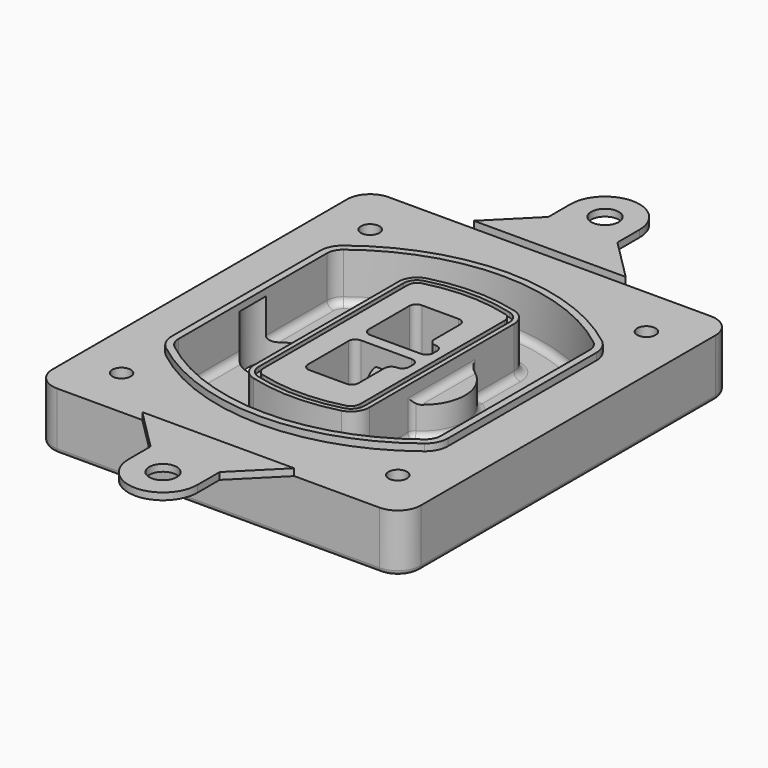
from build123d import *

# Parameters (mm, degrees)
F0_R      = 4
F1_DEPTH  = 25
F2_DEPTH  = 3
F3_DEPTH  = 18
F5_DEPTH  = 21
F6_DEPTH  = 2
F8_DEPTH  = 20
F9_DEPTH  = 16
F10_DEPTH = 25
F7_R      = 6
F7_R_2    = 4
F11_DEPTH = 6
F13_DEPTH = 9
F14_R     = 3
F15_R     = 2
F16_R     = 6
F17_DEPTH = 3


# Not quite as in the source:
# - a feature names something its author has since deleted; it is built from what else it names


with BuildPart() as f1:
    # F0 (on Top) → F1 (new body)
    with BuildSketch(Plane.XY):
        with BuildLine():
            ThreePointArc((-80, -80), (-77.0710678119, -87.0710678119), (-70, -90))
            Line((-70, -90), (70, -90))
            ThreePointArc((70, -90), (77.0710678119, -87.0710678119), (80, -80))
            Line((80, -80), (80, 80))
            ThreePointArc((80, 80), (77.0710678119, 87.0710678119), (70, 90))
            Line((70, 90), (-70, 90))
            ThreePointArc((-70, 90), (-77.0710678119, 87.0710678119), (-80, 80))
            Line((-80, 80), (-80, -80))
        make_face()
        with Locations((-60, -67.5)):
            Circle(F0_R, mode=Mode.SUBTRACT)
        with Locations((60, -67.5)):
            Circle(F0_R, mode=Mode.SUBTRACT)
        with Locations((-60, 67.5)):
            Circle(F0_R, mode=Mode.SUBTRACT)
        with BuildLine():
            ThreePointArc((-64, 40.2934422872), (-62.5820384798, 46.4328484224), (-58.6153846154, 51.3286200352))
            ThreePointArc((-58.6153846154, 51.3286200352), (0, 71.5), (58.6153846154, 51.3286200352))
            ThreePointArc((58.6153846154, 51.3286200352), (62.5820384798, 46.4328484224), (64, 40.2934422872))
            Line((64, 40.2934422872), (64, -40.2934422872))
            ThreePointArc((64, -40.2934422872), (62.5820384798, -46.4328484224), (58.6153846154, -51.3286200352))
            ThreePointArc((58.6153846154, -51.3286200352), (0, -71.5), (-58.6153846154, -51.3286200352))
            ThreePointArc((-58.6153846154, -51.3286200352), (-62.5820384798, -46.4328484224), (-64, -40.2934422872))
            Line((-64, -40.2934422872), (-64, 40.2934422872))
        make_face(mode=Mode.SUBTRACT)
        with Locations((60, 67.5)):
            Circle(F0_R, mode=Mode.SUBTRACT)
        with BuildLine():
            ThreePointArc((58.6153846154, 51.3286200352), (0, 71.5), (-58.6153846154, 51.3286200352))
            ThreePointArc((-58.6153846154, 51.3286200352), (-62.5820384798, 46.4328484224), (-64, 40.2934422872))
            Line((-64, 40.2934422872), (-64, -40.2934422872))
            ThreePointArc((-64, -40.2934422872), (-62.5820384798, -46.4328484224), (-58.6153846154, -51.3286200352))
            ThreePointArc((-58.6153846154, -51.3286200352), (0, -71.5), (58.6153846154, -51.3286200352))
            ThreePointArc((58.6153846154, -51.3286200352), (62.5820384798, -46.4328484224), (64, -40.2934422872))
            Line((64, -40.2934422872), (64, 40.2934422872))
            ThreePointArc((64, 40.2934422872), (62.5820384798, 46.4328484224), (58.6153846154, 51.3286200352))
        make_face()
        with BuildLine():
            Line((-60, -40.2934422872), (-60, 40.2934422872))
            ThreePointArc((-60, 40.2934422872), (-58.9871703427, 44.6787323838), (-56.1538461538, 48.1757121072))
            ThreePointArc((-56.1538461538, 48.1757121072), (0, 67.5), (56.1538461538, 48.1757121072))
            ThreePointArc((56.1538461538, 48.1757121072), (58.9871703427, 44.6787323838), (60, 40.2934422872))
            Line((60, 40.2934422872), (60, -40.2934422872))
            ThreePointArc((60, -40.2934422872), (58.9871703427, -44.6787323838), (56.1538461538, -48.1757121072))
            ThreePointArc((56.1538461538, -48.1757121072), (0, -67.5), (-56.1538461538, -48.1757121072))
            ThreePointArc((-56.1538461538, -48.1757121072), (-58.9871703427, -44.6787323838), (-60, -40.2934422872))
        make_face(mode=Mode.SUBTRACT)
        with BuildLine():
            ThreePointArc((-56.1538461538, 48.1757121072), (-58.9871703427, 44.6787323838), (-60, 40.2934422872))
            Line((-60, 40.2934422872), (-60, -40.2934422872))
            ThreePointArc((-60, -40.2934422872), (-58.9871703427, -44.6787323838), (-56.1538461538, -48.1757121072))
            ThreePointArc((-56.1538461538, -48.1757121072), (0, -67.5), (56.1538461538, -48.1757121072))
            ThreePointArc((56.1538461538, -48.1757121072), (58.9871703427, -44.6787323838), (60, -40.2934422872))
            Line((60, -40.2934422872), (60, 40.2934422872))
            ThreePointArc((60, 40.2934422872), (58.9871703427, 44.6787323838), (56.1538461538, 48.1757121072))
            ThreePointArc((56.1538461538, 48.1757121072), (0, 67.5), (-56.1538461538, 48.1757121072))
        make_face()
        with BuildLine():
            ThreePointArc((54.3076923077, 45.8110311612), (56.2910192399, 43.3631453548), (57, 40.2934422872))
            Line((57, 40.2934422872), (57, -40.2934422872))
            ThreePointArc((57, -40.2934422872), (56.2910192399, -43.3631453548), (54.3076923077, -45.8110311612))
            ThreePointArc((54.3076923077, -45.8110311612), (0, -64.5), (-54.3076923077, -45.8110311612))
            ThreePointArc((-54.3076923077, -45.8110311612), (-56.2910192399, -43.3631453548), (-57, -40.2934422872))
            Line((-57, -40.2934422872), (-57, 40.2934422872))
            ThreePointArc((-57, 40.2934422872), (-56.2910192399, 43.3631453548), (-54.3076923077, 45.8110311612))
            ThreePointArc((-54.3076923077, 45.8110311612), (0, 64.5), (54.3076923077, 45.8110311612))
        make_face(mode=Mode.SUBTRACT)
        with BuildLine():
            Line((57, -40.2934422872), (57, 40.2934422872))
            ThreePointArc((57, 40.2934422872), (56.2910192399, 43.3631453548), (54.3076923077, 45.8110311612))
            ThreePointArc((54.3076923077, 45.8110311612), (0, 64.5), (-54.3076923077, 45.8110311612))
            ThreePointArc((-54.3076923077, 45.8110311612), (-56.2910192399, 43.3631453548), (-57, 40.2934422872))
            Line((-57, 40.2934422872), (-57, -40.2934422872))
            ThreePointArc((-57, -40.2934422872), (-56.2910192399, -43.3631453548), (-54.3076923077, -45.8110311612))
            ThreePointArc((-54.3076923077, -45.8110311612), (0, -64.5), (54.3076923077, -45.8110311612))
            ThreePointArc((54.3076923077, -45.8110311612), (56.2910192399, -43.3631453548), (57, -40.2934422872))
        make_face()
    extrude(amount=-F1_DEPTH)

    # F0 (on Top) → F2 (join)
    with BuildSketch(Plane.XY):
        with BuildLine():
            ThreePointArc((-56.1538461538, 48.1757121072), (-58.9871703427, 44.6787323838), (-60, 40.2934422872))
            Line((-60, 40.2934422872), (-60, -40.2934422872))
            ThreePointArc((-60, -40.2934422872), (-58.9871703427, -44.6787323838), (-56.1538461538, -48.1757121072))
            ThreePointArc((-56.1538461538, -48.1757121072), (0, -67.5), (56.1538461538, -48.1757121072))
            ThreePointArc((56.1538461538, -48.1757121072), (58.9871703427, -44.6787323838), (60, -40.2934422872))
            Line((60, -40.2934422872), (60, 40.2934422872))
            ThreePointArc((60, 40.2934422872), (58.9871703427, 44.6787323838), (56.1538461538, 48.1757121072))
            ThreePointArc((56.1538461538, 48.1757121072), (0, 67.5), (-56.1538461538, 48.1757121072))
        make_face()
        with BuildLine():
            ThreePointArc((54.3076923077, 45.8110311612), (56.2910192399, 43.3631453548), (57, 40.2934422872))
            Line((57, 40.2934422872), (57, -40.2934422872))
            ThreePointArc((57, -40.2934422872), (56.2910192399, -43.3631453548), (54.3076923077, -45.8110311612))
            ThreePointArc((54.3076923077, -45.8110311612), (0, -64.5), (-54.3076923077, -45.8110311612))
            ThreePointArc((-54.3076923077, -45.8110311612), (-56.2910192399, -43.3631453548), (-57, -40.2934422872))
            Line((-57, -40.2934422872), (-57, 40.2934422872))
            ThreePointArc((-57, 40.2934422872), (-56.2910192399, 43.3631453548), (-54.3076923077, 45.8110311612))
            ThreePointArc((-54.3076923077, 45.8110311612), (0, 64.5), (54.3076923077, 45.8110311612))
        make_face(mode=Mode.SUBTRACT)
    extrude(amount=F2_DEPTH)

    # F0 (on Top) → F3 (cut)
    with BuildSketch(Plane.XY):
        with BuildLine():
            Line((57, -40.2934422872), (57, 40.2934422872))
            ThreePointArc((57, 40.2934422872), (56.2910192399, 43.3631453548), (54.3076923077, 45.8110311612))
            ThreePointArc((54.3076923077, 45.8110311612), (0, 64.5), (-54.3076923077, 45.8110311612))
            ThreePointArc((-54.3076923077, 45.8110311612), (-56.2910192399, 43.3631453548), (-57, 40.2934422872))
            Line((-57, 40.2934422872), (-57, -40.2934422872))
            ThreePointArc((-57, -40.2934422872), (-56.2910192399, -43.3631453548), (-54.3076923077, -45.8110311612))
            ThreePointArc((-54.3076923077, -45.8110311612), (0, -64.5), (54.3076923077, -45.8110311612))
            ThreePointArc((54.3076923077, -45.8110311612), (56.2910192399, -43.3631453548), (57, -40.2934422872))
        make_face()
    extrude(amount=-F3_DEPTH, mode=Mode.SUBTRACT)

    # F4 (on face) → F5 (join, through all)
    with BuildSketch(Plane.XY.offset(3)):
        with BuildLine():
            ThreePointArc((-25, -39.2465276821), (-23.3511545998, -44.1109737193), (-19.0842911877, -46.9702398883))
            ThreePointArc((-19.0842911877, -46.9702398883), (0, -49.5), (19.0842911877, -46.9702398883))
            ThreePointArc((19.0842911877, -46.9702398883), (23.3511545998, -44.1109737193), (25, -39.2465276821))
            Line((25, -39.2465276821), (25, 39.2465276821))
            ThreePointArc((25, 39.2465276821), (23.3511545998, 44.1109737193), (19.0842911877, 46.9702398883))
            ThreePointArc((19.0842911877, 46.9702398883), (0, 49.5), (-19.0842911877, 46.9702398883))
            ThreePointArc((-19.0842911877, 46.9702398883), (-23.3511545998, 44.1109737193), (-25, 39.2465276821))
            Line((-25, 39.2465276821), (-25, -39.2465276821))
        make_face()
        with BuildLine():
            ThreePointArc((18.5632183908, 45.0393118368), (21.7633659499, 42.89486221), (23, 39.2465276821))
            Line((23, 39.2465276821), (23, -39.2465276821))
            ThreePointArc((23, -39.2465276821), (21.7633659499, -42.89486221), (18.5632183908, -45.0393118368))
            ThreePointArc((18.5632183908, -45.0393118368), (0, -47.5), (-18.5632183908, -45.0393118368))
            ThreePointArc((-18.5632183908, -45.0393118368), (-21.7633659499, -42.89486221), (-23, -39.2465276821))
            Line((-23, -39.2465276821), (-23, 39.2465276821))
            ThreePointArc((-23, 39.2465276821), (-21.7633659499, 42.89486221), (-18.5632183908, 45.0393118368))
            ThreePointArc((-18.5632183908, 45.0393118368), (0, 47.5), (18.5632183908, 45.0393118368))
        make_face(mode=Mode.SUBTRACT)
        with BuildLine():
            Line((23, -39.2465276821), (23, 39.2465276821))
            ThreePointArc((23, 39.2465276821), (21.7633659499, 42.89486221), (18.5632183908, 45.0393118368))
            ThreePointArc((18.5632183908, 45.0393118368), (0, 47.5), (-18.5632183908, 45.0393118368))
            ThreePointArc((-18.5632183908, 45.0393118368), (-21.7633659499, 42.89486221), (-23, 39.2465276821))
            Line((-23, 39.2465276821), (-23, -39.2465276821))
            ThreePointArc((-23, -39.2465276821), (-21.7633659499, -42.89486221), (-18.5632183908, -45.0393118368))
            ThreePointArc((-18.5632183908, -45.0393118368), (0, -47.5), (18.5632183908, -45.0393118368))
            ThreePointArc((18.5632183908, -45.0393118368), (21.7633659499, -42.89486221), (23, -39.2465276821))
        make_face()
        with BuildLine():
            ThreePointArc((18.0421455939, 43.1083837852), (20.1755772999, 41.6787507007), (21, 39.2465276821))
            Line((21, 39.2465276821), (21, -39.2465276821))
            ThreePointArc((21, -39.2465276821), (20.1755772999, -41.6787507007), (18.0421455939, -43.1083837852))
            ThreePointArc((18.0421455939, -43.1083837852), (0, -45.5), (-18.0421455939, -43.1083837852))
            ThreePointArc((-18.0421455939, -43.1083837852), (-20.1755772999, -41.6787507007), (-21, -39.2465276821))
            Line((-21, -39.2465276821), (-21, 39.2465276821))
            ThreePointArc((-21, 39.2465276821), (-20.1755772999, 41.6787507007), (-18.0421455939, 43.1083837852))
            ThreePointArc((-18.0421455939, 43.1083837852), (0, 45.5), (18.0421455939, 43.1083837852))
        make_face(mode=Mode.SUBTRACT)
        with BuildLine():
            Line((21, -39.2465276821), (21, 39.2465276821))
            ThreePointArc((21, 39.2465276821), (20.1755772999, 41.6787507007), (18.0421455939, 43.1083837852))
            ThreePointArc((18.0421455939, 43.1083837852), (0, 45.5), (-18.0421455939, 43.1083837852))
            ThreePointArc((-18.0421455939, 43.1083837852), (-20.1755772999, 41.6787507007), (-21, 39.2465276821))
            Line((-21, 39.2465276821), (-21, -39.2465276821))
            ThreePointArc((-21, -39.2465276821), (-20.1755772999, -41.6787507007), (-18.0421455939, -43.1083837852))
            ThreePointArc((-18.0421455939, -43.1083837852), (0, -45.5), (18.0421455939, -43.1083837852))
            ThreePointArc((18.0421455939, -43.1083837852), (20.1755772999, -41.6787507007), (21, -39.2465276821))
        make_face()
        with BuildLine():
            Line((-8, -2.5), (14, -2.5))
            ThreePointArc((14, -2.5), (16.1213203436, -3.3786796564), (17, -5.5))
            Line((17, -5.5), (17, -7.5))
            ThreePointArc((17, -7.5), (16.1213203436, -9.6213203436), (14, -10.5))
            ThreePointArc((14, -10.5), (11.8786796564, -11.3786796564), (11, -13.5))
            Line((11, -13.5), (11, -27.5))
            ThreePointArc((11, -27.5), (10.1213203436, -29.6213203436), (8, -30.5))
            Line((8, -30.5), (-8, -30.5))
            ThreePointArc((-8, -30.5), (-10.1213203436, -29.6213203436), (-11, -27.5))
            Line((-11, -27.5), (-11, -5.5))
            ThreePointArc((-11, -5.5), (-10.1213203436, -3.3786796564), (-8, -2.5))
        make_face(mode=Mode.SUBTRACT)
        with BuildLine():
            ThreePointArc((-8, 2.5), (-10.1213203436, 3.3786796564), (-11, 5.5))
            Line((-11, 5.5), (-11, 27.5))
            ThreePointArc((-11, 27.5), (-10.1213203436, 29.6213203436), (-8, 30.5))
            Line((-8, 30.5), (8, 30.5))
            ThreePointArc((8, 30.5), (10.1213203436, 29.6213203436), (11, 27.5))
            Line((11, 27.5), (11, 13.5))
            ThreePointArc((11, 13.5), (11.8786796564, 11.3786796564), (14, 10.5))
            ThreePointArc((14, 10.5), (16.1213203436, 9.6213203436), (17, 7.5))
            Line((17, 7.5), (17, 5.5))
            ThreePointArc((17, 5.5), (16.1213203436, 3.3786796564), (14, 2.5))
            Line((14, 2.5), (-8, 2.5))
        make_face(mode=Mode.SUBTRACT)
    extrude(amount=-F5_DEPTH)

    # F4 (on face) → F6 (cut)
    with BuildSketch(Plane.XY.offset(3)):
        with BuildLine():
            Line((23, -39.2465276821), (23, 39.2465276821))
            ThreePointArc((23, 39.2465276821), (21.7633659499, 42.89486221), (18.5632183908, 45.0393118368))
            ThreePointArc((18.5632183908, 45.0393118368), (0, 47.5), (-18.5632183908, 45.0393118368))
            ThreePointArc((-18.5632183908, 45.0393118368), (-21.7633659499, 42.89486221), (-23, 39.2465276821))
            Line((-23, 39.2465276821), (-23, -39.2465276821))
            ThreePointArc((-23, -39.2465276821), (-21.7633659499, -42.89486221), (-18.5632183908, -45.0393118368))
            ThreePointArc((-18.5632183908, -45.0393118368), (0, -47.5), (18.5632183908, -45.0393118368))
            ThreePointArc((18.5632183908, -45.0393118368), (21.7633659499, -42.89486221), (23, -39.2465276821))
        make_face()
        with BuildLine():
            ThreePointArc((18.0421455939, 43.1083837852), (20.1755772999, 41.6787507007), (21, 39.2465276821))
            Line((21, 39.2465276821), (21, -39.2465276821))
            ThreePointArc((21, -39.2465276821), (20.1755772999, -41.6787507007), (18.0421455939, -43.1083837852))
            ThreePointArc((18.0421455939, -43.1083837852), (0, -45.5), (-18.0421455939, -43.1083837852))
            ThreePointArc((-18.0421455939, -43.1083837852), (-20.1755772999, -41.6787507007), (-21, -39.2465276821))
            Line((-21, -39.2465276821), (-21, 39.2465276821))
            ThreePointArc((-21, 39.2465276821), (-20.1755772999, 41.6787507007), (-18.0421455939, 43.1083837852))
            ThreePointArc((-18.0421455939, 43.1083837852), (0, 45.5), (18.0421455939, 43.1083837852))
        make_face(mode=Mode.SUBTRACT)
    extrude(amount=-F6_DEPTH, mode=Mode.SUBTRACT)

    # F7 (on face) → F8 (join)
    with BuildSketch(Plane(origin=(0, 0, -25), x_dir=(1, 0, 0), z_dir=(0, 0, -1))):
        with BuildLine():
            ThreePointArc((3.28842436, 0), (16.7567035675, 13.4682792075), (30.224982775, 0))
            Line((30.224982775, 0), (35.224982775, 0))
            ThreePointArc((35.224982775, 0), (16.7567035675, 18.4682792075), (-1.71157564, 0))
            Line((-1.71157564, 0), (3.28842436, 0))
        make_face()
        with BuildLine():
            Line((3.28842436, 0), (30.224982775, 0))
            ThreePointArc((30.224982775, 0), (16.7567035675, 13.4682792075), (3.28842436, 0))
        make_face()
        with BuildLine():
            ThreePointArc((3.28842436, 0), (16.7567035675, -13.4682792075), (30.224982775, 0))
            Line((30.224982775, 0), (3.28842436, 0))
        make_face()
        with BuildLine():
            Line((35.224982775, 0), (30.224982775, 0))
            ThreePointArc((30.224982775, 0), (16.7567035675, -13.4682792075), (3.28842436, 0))
            Line((3.28842436, 0), (-1.71157564, 0))
            ThreePointArc((-1.71157564, 0), (16.7567035675, -18.4682792075), (35.224982775, 0))
        make_face()
    extrude(amount=-F8_DEPTH)

    # F7 (on face) → F9 (cut)
    with BuildSketch(Plane(origin=(0, 0, -25), x_dir=(1, 0, 0), z_dir=(0, 0, -1))):
        with BuildLine():
            Line((3.28842436, 0), (30.224982775, 0))
            ThreePointArc((30.224982775, 0), (16.7567035675, 13.4682792075), (3.28842436, 0))
        make_face()
        with BuildLine():
            ThreePointArc((3.28842436, 0), (16.7567035675, -13.4682792075), (30.224982775, 0))
            Line((30.224982775, 0), (3.28842436, 0))
        make_face()
    extrude(amount=-F9_DEPTH, mode=Mode.SUBTRACT)

    # F7 (on face) → F10 (cut)
    with BuildSketch(Plane(origin=(0, 0, -25), x_dir=(1, 0, 0), z_dir=(0, 0, -1))):
        with BuildLine():
            Line((-59.0318229325, 0), (-32.0952645175, 0))
            ThreePointArc((-32.0952645175, 0), (-45.563543725, 13.4682792075), (-59.0318229325, 0))
        make_face()
        with BuildLine():
            ThreePointArc((-59.0318229325, 0), (-45.563543725, -13.4682792075), (-32.0952645175, 0))
            Line((-32.0952645175, 0), (-59.0318229325, 0))
        make_face()
    extrude(amount=-F10_DEPTH, mode=Mode.SUBTRACT)

    # F7 (on face) → F11 (cut)
    with BuildSketch(Plane(origin=(0, 0, -25), x_dir=(1, 0, 0), z_dir=(0, 0, -1))):
        with Locations((60, -67.5)):
            Circle(F7_R)
        with Locations((60, -67.5)):
            Circle(F7_R_2, mode=Mode.SUBTRACT)
        with Locations((-60, -67.5)):
            Circle(F7_R)
        with Locations((-60, -67.5)):
            Circle(F7_R_2, mode=Mode.SUBTRACT)
        with Locations((-60, 67.5)):
            Circle(F7_R)
        with Locations((-60, 67.5)):
            Circle(F7_R_2, mode=Mode.SUBTRACT)
        with Locations((60, 67.5)):
            Circle(F7_R)
        with Locations((60, 67.5)):
            Circle(F7_R_2, mode=Mode.SUBTRACT)
    extrude(amount=-F11_DEPTH, mode=Mode.SUBTRACT)

    # F12 (on face) → F13 (cut, through all)
    with BuildSketch(Plane(origin=(0, 0, -9), x_dir=(1, 0, 0), z_dir=(0, 0, -1))):
        with BuildLine():
            Line((11, 13.5), (11, 17.5481537753))
            ThreePointArc((11, 17.5481537753), (2.5696536419, 11.8239143813), (-1.5415842455, 2.5))
            Line((-1.5415842455, 2.5), (3.5224848595, 2.5))
            ThreePointArc((3.5224848595, 2.5), (6.1857188154, 8.3455872281), (11.2536447004, 12.2927168648))
            ThreePointArc((11.2536447004, 12.2927168648), (11.0640958889, 12.8831798879), (11, 13.5))
        make_face()
        with BuildLine():
            ThreePointArc((11.2536447004, -12.2927168648), (6.1857188154, -8.3455872281), (3.5224848595, -2.5))
            Line((3.5224848595, -2.5), (-1.5415842455, -2.5))
            ThreePointArc((-1.5415842455, -2.5), (2.5696536419, -11.8239143813), (11, -17.5481537753))
            Line((11, -17.5481537753), (11, -13.5))
            ThreePointArc((11, -13.5), (11.0640958889, -12.8831798879), (11.2536447004, -12.2927168648))
        make_face()
        with BuildLine():
            ThreePointArc((11.2536447004, 12.2927168648), (6.1857188154, 8.3455872281), (3.5224848595, 2.5))
            Line((3.5224848595, 2.5), (14, 2.5))
            ThreePointArc((14, 2.5), (16.1213203436, 3.3786796564), (17, 5.5))
            Line((17, 5.5), (17, 7.5))
            ThreePointArc((17, 7.5), (16.1213203436, 9.6213203436), (14, 10.5))
            ThreePointArc((14, 10.5), (12.3601599782, 10.9878446101), (11.2536447004, 12.2927168648))
        make_face()
        with BuildLine():
            Line((14, -2.5), (3.5224848595, -2.5))
            ThreePointArc((3.5224848595, -2.5), (6.1857188154, -8.3455872281), (11.2536447004, -12.2927168648))
            ThreePointArc((11.2536447004, -12.2927168648), (12.3601599782, -10.9878446101), (14, -10.5))
            ThreePointArc((14, -10.5), (16.1213203436, -9.6213203436), (17, -7.5))
            Line((17, -7.5), (17, -5.5))
            ThreePointArc((17, -5.5), (16.1213203436, -3.3786796564), (14, -2.5))
        make_face()
    extrude(amount=F13_DEPTH, mode=Mode.SUBTRACT)

    # F14
    f14_edges = [f1.edges().sort_by_distance(p)[0] for p in [
        (-57, -23.703476, -18),
        (-57, 23.703476, -18),
        (25, 0, -5),
        (25, 16.526506, -11.5),
        (25, -16.526506, -11.5),
        (25, -27.886517, -18),
        (35.224983, 0, -18),
    ]]
    fillet(f14_edges, radius=F14_R)

    # F15
    f15_edges = [f1.edges().sort_by_distance(p)[0] for p in [
        (0, -90, -25),
    ]]
    fillet(f15_edges, radius=F15_R)


with BuildPart() as f17:
    # F16 (on face) → F17 (new body, through all)
    with BuildSketch(Plane.XY):
        with BuildLine():
            Line((-15, 108), (-33, 90))
            Line((-33, 90), (33, 90))
            Line((33, 90), (15, 108))
            Line((15, 108), (15, 120))
            ThreePointArc((15, 120), (0, 135), (-15, 120))
            Line((-15, 120), (-15, 108))
        make_face()
        with Locations((0, 120)):
            Circle(F16_R, mode=Mode.SUBTRACT)
    extrude(amount=F17_DEPTH)


with BuildPart() as f17b:
    # F16 (on face) → F17, piece 2 (new body, through all)
    with BuildSketch(Plane.XY):
        with BuildLine():
            Line((33, -90), (-33, -90))
            Line((-33, -90), (-15, -108))
            Line((-15, -108), (-15, -120))
            ThreePointArc((-15, -120), (0, -135), (15, -120))
            Line((15, -120), (15, -108))
            Line((15, -108), (33, -90))
        make_face()
        with Locations((0, -120)):
            Circle(F16_R, mode=Mode.SUBTRACT)
    extrude(amount=F17_DEPTH)


solid = Compound([f1.part, f17.part, f17b.part])
